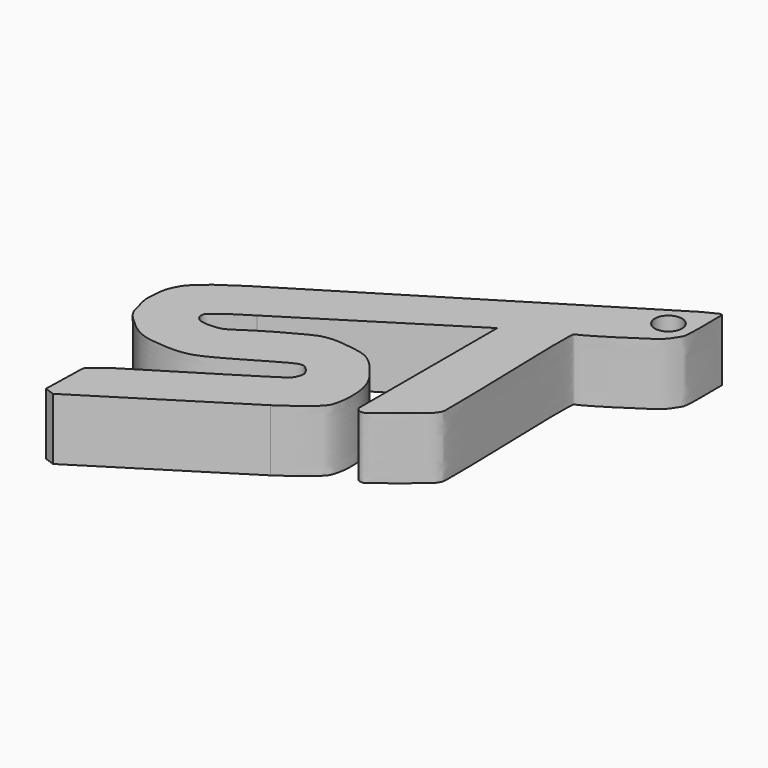
from build123d import *

# Parameters (mm, degrees)
F1_DEPTH = 6.35
F3_D     = 2.794


with BuildPart() as f1:
    # F0 (on Top) → F1 (new body)
    with BuildSketch(Plane.XY):
        with BuildLine():
            Line((39.4817653725, -37.0192130655), (39.3676378211, -41.6417355957))
            Line((39.3676378211, -41.6417355957), (40.3558458004, -42.0050450858))
            Line((40.3558458004, -42.0050450858), (55.2362861492, -32.6425464452))
            add(Edge.make_bspline(
                [(44.6505507136, -21.1328643933), (43.8894052591, -21.594743934), (42.5955364359, -22.3798915484), (41.5978946674, -23.2154812849), (41.2567670852, -23.4456688432), (41.132849027, -23.7969929094), (41.1324892762, -24.0451827411), (41.2346934987, -24.311347919), (41.364111181, -24.4582967657), (41.5888940208, -24.6637994238), (41.8062818008, -24.7549946052), (42.2324095062, -24.8052103975), (42.6009533355, -24.8510306386), (43.1920548585, -24.8009051339), (44.1276926829, -24.7279275276), (45.8496310644, -23.3615463856), (49.9593339535, -21.1031665183), (51.0277793958, -20.6686062974), (52.4590086434, -20.5095061466), (54.1037747992, -20.7632235807), (55.6770163425, -20.9996288915), (56.821448891, -21.9098698969), (57.5403873531, -22.779150825), (58.5854624812, -24.0430171052), (59.2844131497, -25.641827004), (59.3395727511, -27.3870846743), (59.3044495058, -28.2258904909), (59.1313004465, -29.0040529813), (59.019643645, -29.5137641111), (58.5782200458, -30.0873099325), (57.5333588739, -31.0406933356), (56.0904159459, -32.0469229562), (55.2362861492, -32.6425464452)],
                knots=[0, 0, 0, 0, 0.0525837686, 0.0893869869, 0.1098139196, 0.1291325162, 0.1457822037, 0.162988682, 0.1778842391, 0.195757994, 0.2120029538, 0.2333517062, 0.2537786373, 0.2787724187, 0.3090618218, 0.3589650655, 0.430972174, 0.4670530399, 0.5052884931, 0.5485701802, 0.5903570256, 0.6294282656, 0.6647527096, 0.7067798515, 0.7511104677, 0.7944348039, 0.825097015, 0.8540849852, 0.8777055221, 0.9046658963, 0.9435683165, 1, 1, 1, 1], degree=3))
            Line((44.6505507136, -21.1328643933), (60.7135896979, -11.0262965009))
            Line((60.7135896979, -11.0262965009), (61.0709478256, -10.8014533574))
            Line((61.0709478256, -10.8014533574), (61.0709478256, -28.2584297099))
            add(Edge.make_bspline(
                [(61.0709478256, -28.2584297099), (61.0595833019, -28.3555682228), (61.0361501708, -28.5558634201), (61.2198413396, -28.8562441229), (61.5096848503, -29.0188554179), (61.9204299983, -29.0129140073), (62.3636308245, -28.7066703031), (65.3280330283, -26.3419064772), (65.999965611, -25.7471929521), (66.4092392446, -25.4073957503), (66.6387670672, -24.9574692516), (66.9682161496, -24.7469319366), (66.2223671024, -7.8724936683), (66.639592862, -7.7454340397), (67.3075611468, -7.5367304169), (72.2762985848, -4.3500027542), (72.6834717789, -3.9186439743), (73.1217094854, -3.4414147688), (73.4898702317, -2.7590605685), (73.8531650458, -2.3805649258), (73.7019838484, 2.0398269878), (73.7581018067, 2.1415128091), (73.7226334429, 2.2932026392), (73.5988568521, 2.297308914), (73.4939755113, 2.2968938237), (73.4440039525, 2.2831555828)],
                knots=[0, 0, 0, 0, 0.0223820703, 0.0461508113, 0.0697615635, 0.0941666107, 0.1249427412, 0.2056352141, 0.2468950841, 0.2757139206, 0.3022841671, 0.3312767984, 0.5003028796, 0.5207871087, 0.5541905771, 0.6549044403, 0.6893617869, 0.7210764276, 0.7559321916, 0.7891031447, 0.8746725905, 0.8900704558, 0.9040170523, 0.9177184702, 0.9342754996, 0.9342754996, 0.9342754996, 0.9342754996], degree=3))
            add(Edge.make_bspline(
                [(73.3087232087, 2.215904887), (73.3538167899, 2.2383217856), (73.3989103712, 2.2607386842), (73.4440039525, 2.2831555828)],
                knots=[1.4000692571, 1.4000692571, 1.4000692571, 1.4000692571, 1.5511438603, 1.5511438603, 1.5511438603, 1.5511438603], degree=3))
            add(Edge.make_bspline(
                [(72.0550220142, 1.5926655754), (72.4729224123, 1.8004120126), (72.8908228105, 2.0081584498), (73.3087232087, 2.215904887)],
                knots=[0, 0, 0, 0, 1.4000692571, 1.4000692571, 1.4000692571, 1.4000692571], degree=3))
            Line((72.0550220142, 1.5926655754), (40.8347721825, -17.6163617149))
            add(Edge.make_bspline(
                [(40.8347721825, -17.6163617149), (39.8689293975, -18.2563133661), (38.5476931743, -19.1317429037), (38.2457886692, -19.4180780584), (37.8709121737, -19.7307314041), (37.4450231839, -20.113852652), (36.8831177301, -20.620905643), (36.4747703446, -21.3081182265), (36.1729086727, -21.941030601), (36.0325110796, -22.4885651887), (35.9328206683, -23.1587767462), (35.8992244224, -24.0325904771), (35.8788641312, -24.5237365635), (35.9965011884, -25.079002316), (36.224985635, -25.9992294138), (36.5196289869, -27.0955534999), (37.5872292158, -28.1545601487), (39.2775107604, -29.6169682126), (41.6513761522, -29.9432728243), (44.3782963168, -30.0271412886), (46.6141536812, -28.929305647), (49.6508476137, -27.2139041305), (52.1611038389, -25.6522317715), (53.020313778, -25.526641351), (53.4818227455, -25.8881862026), (53.8198805798, -26.3333429487), (54.0473119149, -26.8173388111), (53.6270320713, -27.7961403968), (53.018467696, -28.2758716997), (42.0850035568, -35.0652841461), (40.9475966137, -35.7020198511), (39.9743791138, -36.5765512781), (39.4817653725, -37.0192130655)],
                knots=[0, 0, 0, 0, 0.0485374277, 0.0663973564, 0.0858018373, 0.1079781586, 0.1331840138, 0.159255599, 0.1834372474, 0.2049483335, 0.2290436743, 0.2561779586, 0.2763870825, 0.2977556304, 0.325977813, 0.3564719507, 0.3916594354, 0.4344224879, 0.4791991963, 0.5263703788, 0.5717086482, 0.6271273328, 0.676741596, 0.7016018974, 0.7226200165, 0.7441991217, 0.7648483615, 0.7919826461, 0.82045488, 0.9232858051, 0.9611695571, 1, 1, 1, 1], degree=3))
        make_face()
    extrude(amount=F1_DEPTH)

    # F3 (through all)
    with Locations(Plane.XY.offset(6.35)):
        with Locations((71.3086277246, -1.6019018367)):
            Hole(F3_D / 2)


solid = f1.part
